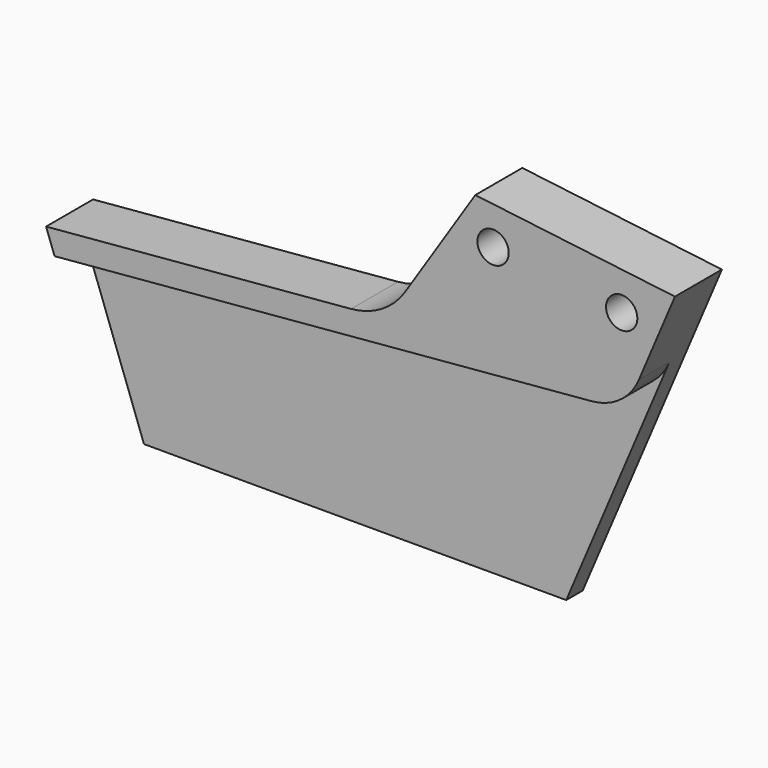
from build123d import *

# Parameters (mm, degrees)
F0_R     = 4.2291
F1_DEPTH = 15.875
F3_DEPTH = 10.3124


# Not quite as in the source:
# - a feature of the source that left no trace in its solid (it failed there, or was rolled back) is left out


with BuildPart() as f1:
    # F0 (on Front) → F1 (new body)
    with BuildSketch(Plane.XZ):
        with BuildLine():
            Line((14.3947540456, 8.4944370214), (-39.560838545, 15.1193507659))
            Line((-39.560838545, 15.1193507659), (-58.5532654186, -14.1264219546))
            ThreePointArc((-58.5532654186, -14.1264219546), (-64.8424818087, -20.1998476249), (-73.1576066321, -22.9015954566))
            Line((-73.1576066321, -22.9015954566), (-155.5821148258, -30.1128055203))
            Line((-155.5821148258, -30.1128055203), (-137.3697370291, -80.1509022713))
            Line((-137.3697370291, -80.1509022713), (-23.2329600585, -80.1509022713))
            Line((-23.2329600585, -80.1509022713), (14.3947540456, 8.4944370214))
        make_face()
        with Locations((-34.7655170351, 4.2686687437)):
            Circle(F0_R, mode=Mode.SUBTRACT)
        Circle(F0_R, mode=Mode.SUBTRACT)
    extrude(amount=F1_DEPTH)

    # F2 (on face) → F3 (cut)
    with BuildSketch(Plane.XZ.offset(15.875)):
        with BuildLine():
            Line((-8.0578011567, -23.7078415676), (-153.2887042884, -36.4138991852))
            Line((-153.2887042884, -36.4138991852), (-137.3697370291, -80.1509022713))
            Line((-137.3697370291, -80.1509022713), (-23.2329600585, -80.1509022713))
            Line((-23.2329600585, -80.1509022713), (4.6424392905, -14.4805767668))
            ThreePointArc((4.6424392905, -14.4805767668), (-0.4282074312, -20.8552533629), (-8.0578011567, -23.7078415676))
        make_face()
    extrude(amount=-F3_DEPTH, mode=Mode.SUBTRACT)


solid = f1.part
